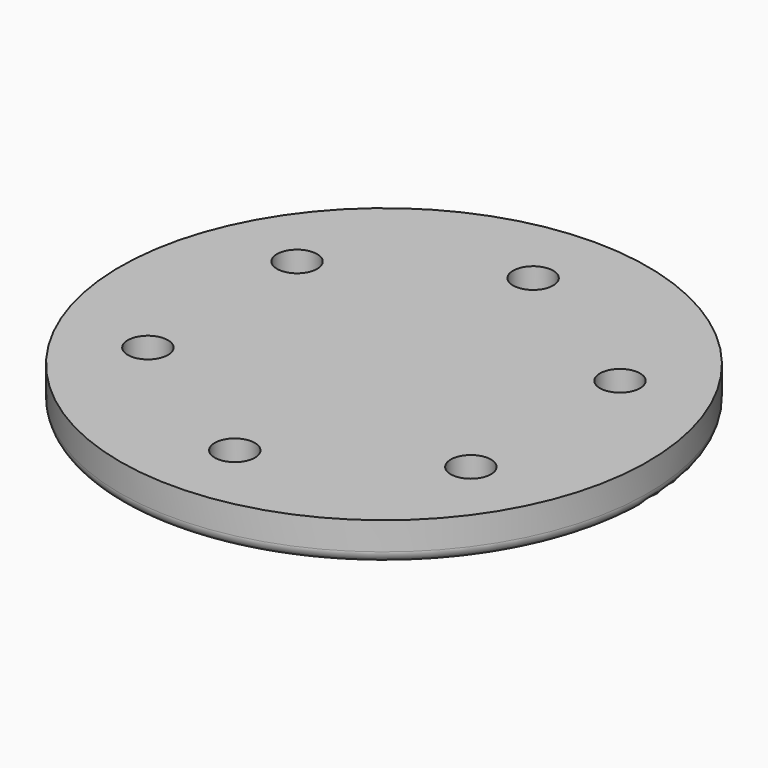
from build123d import *

# Parameters (mm, degrees)
F2_SIZE2        = 2
F2_SIZE         = 2
F3_R            = 7
F4_DEPTH        = 25
F4_COPIES_COUNT = 6


# Not quite as in the source:
# - a pattern or mirror of a feature is missing from the dataset's text; its kind, count and spacing are read off the source's solid


with BuildPart() as f1:
    # F0 (on Right) → F1 (revolve)
    with BuildSketch(Plane.YZ):
        with BuildLine():
            Line((92, 16), (0, 16))
            Line((0, 16), (0, 8))
            Line((0, 8), (43, 8))
            ThreePointArc((43, 8), (44.4142135624, 7.4142135624), (45, 6))
            Line((45, 6), (45, 0))
            Line((45, 0), (80, 0))
            Line((80, 0), (89.0352761804, 2.4209949559))
            ThreePointArc((89.0352761804, 2.4209949559), (91.1734133612, 3.8496525451), (92, 6.2846982611))
            Line((92, 6.2846982611), (92, 16))
        make_face()
    revolve(axis=Axis((0, 0, 0.8759116049), (0, 0, -1)))

    # F2
    f2_edges = [f1.edges().sort_by_distance(p)[0] for p in [
        (0, -45, 0),
    ]]
    chamfer(f2_edges, length=F2_SIZE, length2=F2_SIZE2)

    # F3 (on face) → F4 (cut)
    with BuildSketch(Plane(origin=(0, 0, 0), x_dir=(1, 0, 0), z_dir=(0, 0, -1))):
        with Locations((0, 65)):
            Circle(F3_R)
    f4 = extrude(amount=-F4_DEPTH, mode=Mode.SUBTRACT)

    # F4_copies: F4 ×6 about axis
    f4_copies_axis = Axis((0, 0, 0), (0, 0, 1))
    for i in range(1, F4_COPIES_COUNT):
        add(f4.rotate(f4_copies_axis, i * 360 / F4_COPIES_COUNT), mode=Mode.SUBTRACT)


solid = f1.part
